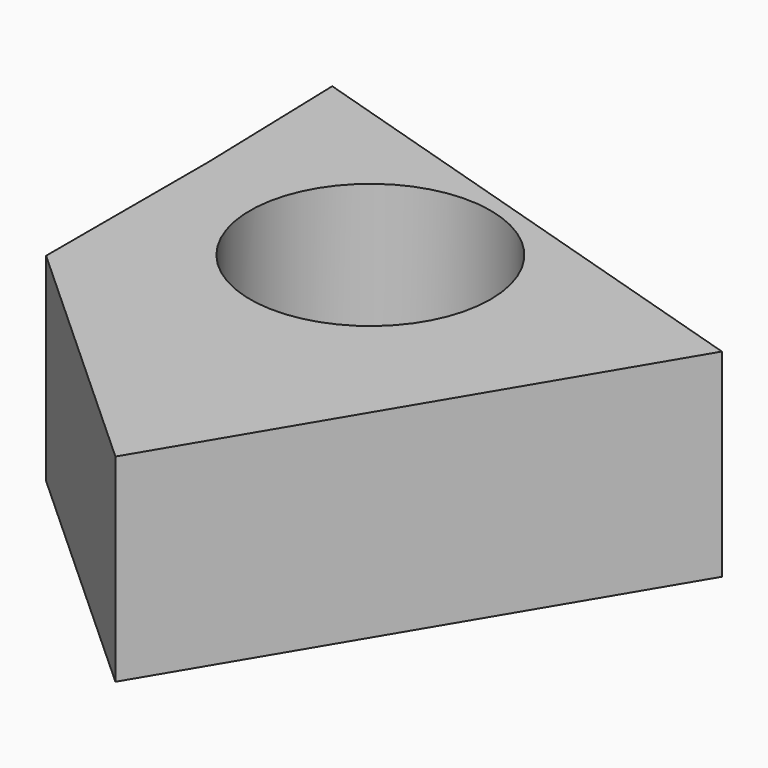
from build123d import *

# Parameters (mm, degrees)
F0_R     = 15.4075582886
F1_DEPTH = 25.4


# Not quite as in the source:
# - a feature of the source that left no trace in its solid (it failed there, or was rolled back) is left out


with BuildPart() as f1:
    # F0 (on Top) → F1 (new body)
    with BuildSketch(Plane.XY):
        Polygon((-33.1784598529, 76.1930122972), (-32.5912311673, 55.6621290743), (-32.5912311673, 29.6373665333), (0, 0), (33.1595037133, 55.6621290743), align=None)
        with Locations((-7.3677506298, 50.0328727067)):
            Circle(F0_R, mode=Mode.SUBTRACT)
    extrude(amount=F1_DEPTH)


solid = f1.part
